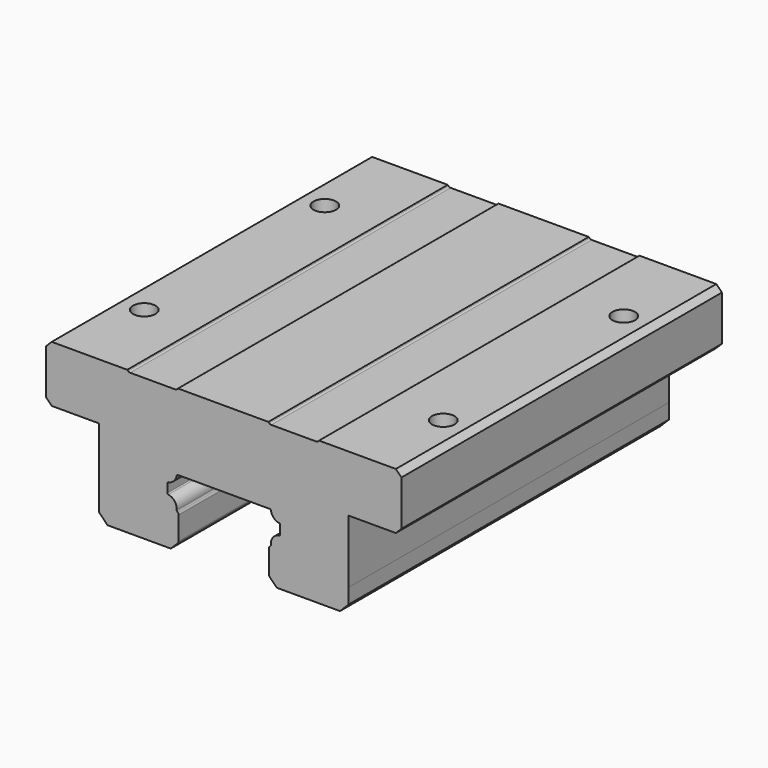
from build123d import *

# Parameters (mm, degrees)
F1_DEPTH = 71
F3_D     = 4


# Not quite as in the source:
# - ends of sketch curves that miss each other by under 0.0002 mm in the source are joined


with BuildPart() as f1:
    # F0 (on Front) → F1 (new body)
    with BuildSketch(Plane.XZ):
        with BuildLine():
            Line((8.1618498422, -10.3647895785), (9.4053820611, -11.6083214649))
            Line((9.4053820611, -11.6083214649), (9.415382064, -11.6183214649))
            Line((9.415382064, -11.6183214649), (20.6153802021, -11.6183214651))
            Line((20.6153802021, -11.6183214651), (22.165411006, -10.0682906612))
            Line((22.165411006, -10.0682906612), (22.1654110059, -7.3944052326))
            Line((22.1654110059, -7.3944052326), (22.1654110059, 3.7817118842))
            Line((22.1654110059, 3.7817118842), (30.0405793841, 3.7817118842))
            Line((30.0405793841, 3.7817118842), (30.515407573, 3.7817104728))
            Line((30.515407573, 3.7817104728), (31.5154075725, 4.7816793802))
            Line((31.5154075725, 4.7816793802), (31.5153703792, 12.7817118841))
            Line((31.5153703792, 12.7817118841), (30.5153417686, 13.7816508489))
            Line((30.5153417686, 13.7816508489), (16.9153093619, 13.7816508489))
            Line((16.9153093619, 13.7816508489), (16.7618646746, 13.6281611659))
            ThreePointArc((16.7618646746, 13.6281611659), (16.5996530095, 13.5197747929), (16.4083113037, 13.4817145544))
            Line((16.4083113037, 13.4817145544), (8.422430452, 13.4817145544))
            ThreePointArc((8.422430452, 13.4817145544), (8.2310887291, 13.5197747818), (8.0688770472, 13.6281611561))
            Line((8.0688770472, 13.6281611561), (7.9153584589, 13.7816508489))
            Line((7.9153584589, 13.7816508489), (-8.0846315282, 13.7816508491))
            Line((-8.0846315282, 13.7816508491), (-8.2381152983, 13.628161166))
            ThreePointArc((-8.2381152983, 13.628161166), (-8.4003269909, 13.5197747816), (-8.5916687288, 13.4817145545))
            Line((-8.5916687288, 13.4817145545), (-16.5775495805, 13.4817145545))
            ThreePointArc((-16.5775495805, 13.4817145545), (-16.7688912713, 13.5197747934), (-16.9311029256, 13.6281611562))
            Line((-16.9311029256, 13.6281611562), (-17.0845685953, 13.7816508491))
            Line((-17.0845685953, 13.7816508491), (-30.4846162694, 13.7816508492))
            Line((-30.4846162694, 13.7816508492), (-31.4846296209, 12.7816374978))
            Line((-31.4846296209, 12.7816374978), (-31.4846296209, 4.7816793804))
            Line((-31.4846296209, 4.7816793804), (-30.4846296214, 3.781710473))
            Line((-30.4846296214, 3.781710473), (-30.0098014316, 3.7817118844))
            Line((-30.0098014316, 3.7817118844), (-22.1346330541, 3.781710473))
            Line((-22.1346330541, 3.781710473), (-22.1346330541, -7.3944052328))
            Line((-22.1346330541, -7.3944052328), (-22.134633054, -10.068299435))
            Line((-22.134633054, -10.068299435), (-20.5846110242, -11.6183214649))
            Line((-20.5846110242, -11.6183214649), (-9.3846416371, -11.618321465))
            Line((-9.3846416371, -11.618321465), (-9.3746416371, -11.6083214649))
            Line((-9.3746416371, -11.6083214649), (-8.1310434239, -10.3647232516))
            ThreePointArc((-8.1310434239, -10.3647232516), (-8.0226570482, -10.2025115772), (-7.9845968145, -10.011169861))
            Line((-7.9845968145, -10.011169861), (-7.9845968145, -5.9254873742))
            ThreePointArc((-7.9845968145, -5.9254873742), (-8.0226567217, -5.7341464462), (-8.1310422173, -5.5719351901))
            Line((-8.1310422173, -5.5719351901), (-8.2697056959, -5.4332707651))
            ThreePointArc((-8.2697056959, -5.4332707651), (-8.3164840652, -5.3595306247), (-8.3273828922, -5.2728874501))
            ThreePointArc((-8.3273828922, -5.2728874501), (-8.6904695936, -4.0063582713), (-9.8182893525, -3.3252190015))
            ThreePointArc((-9.8182893525, -3.3252190015), (-9.9374803464, -3.2570419887), (-9.9846168416, -3.1280739736))
            Line((-9.9846168416, -3.1280739736), (-9.9846168416, -1.6015777605))
            ThreePointArc((-9.9846168416, -1.6015777605), (-9.9374803464, -1.4726097454), (-9.8182893525, -1.4044327326))
            ThreePointArc((-9.8182893525, -1.4044327326), (-8.8323144095, -0.8871586543), (-8.3383526746, 0.1106994843))
            ThreePointArc((-8.3383526746, 0.1106994843), (-8.2712261249, 0.2330065304), (-8.1404708137, 0.2816689983))
            Line((-8.1404708137, 0.2816689983), (8.1712371304, 0.2816689983))
            ThreePointArc((8.1712371304, 0.2816689983), (8.3019924416, 0.2330065304), (8.3691189913, 0.1106994843))
            ThreePointArc((8.3691189913, 0.1106994843), (8.8630871156, -0.8871651956), (9.8490736962, -1.4044358116))
            ThreePointArc((9.8490736962, -1.4044358116), (9.968266036, -1.4726123905), (10.0154031856, -1.6015811811))
            Line((10.0154031856, -1.6015811811), (10.0154031856, -3.1280705531))
            ThreePointArc((10.0154031856, -3.1280705531), (9.968266036, -3.2570393436), (9.8490736962, -3.3252159226))
            ThreePointArc((9.8490736962, -3.3252159226), (8.7212476918, -4.0063428806), (8.3581472677, -5.2728670656))
            ThreePointArc((8.3581472677, -5.2728670656), (8.3472477253, -5.3595093685), (8.3004693733, -5.4332486014))
            Line((8.3004693733, -5.4332486014), (8.161849795, -5.5718681798))
            ThreePointArc((8.161849795, -5.5718681798), (8.0534634193, -5.7340798542), (8.0154031856, -5.9254215704))
            Line((8.0154031856, -5.9254215704), (8.0154031855, -10.0112361406))
            ThreePointArc((8.0154031855, -10.0112361406), (8.0534634321, -10.2025778877), (8.1618498422, -10.3647895785))
        make_face()
    extrude(amount=F1_DEPTH)

    # F3 (through all)
    with Locations(Plane(origin=(0, 0, 0.2816689983), x_dir=(1, 0, 0), z_dir=(0, 0, -1))):
        with Locations((-26.4846296209, 55.5), (26.5153703791, 55.5), (26.5153703791, 15.5), (-26.4846296209, 15.5)):
            Hole(F3_D / 2)


solid = f1.part
